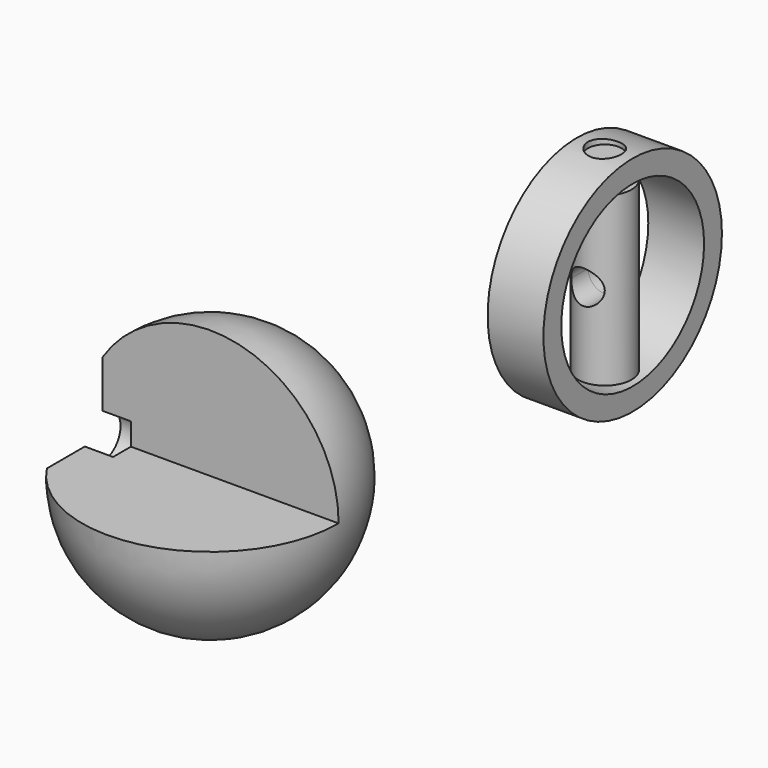
from build123d import *

# Parameters (mm, degrees)
F4_ANGLE       = 270
F5_R           = 10
F5_R_2         = 8
F6_DEPTH       = 5
F8_DEPTH       = 11
F8_DEPTH_BACK  = 25
F11_DEPTH      = 7.5
F11_DEPTH_BACK = 7.5
F12_DEPTH      = 4
F12_DEPTH_BACK = 4
F13_R          = 1.5
F14_DEPTH      = 2
F15_R          = 1.5
F16_DEPTH      = 2


# Not quite as in the source:
# - the program builds the solid bodies; features that only make, move or delete a surface that nothing else refers to are left out


with BuildPart() as f4:
    # F3 (on Front) → F4 (revolve)
    with BuildSketch(Plane.XZ):
        with BuildLine():
            Line((-7.119815331, 0), (11.5, 0))
            ThreePointArc((11.5, 0), (3.2585484641, 11.0286835981), (-9.6533672882, 6.25))
            Line((-9.6533672882, 6.25), (-9.6533672882, 2))
            Line((-9.6533672882, 2), (-7.119815331, 2))
            Line((-7.119815331, 2), (-7.119815331, 0))
        make_face()
    revolve(axis=Axis((-0.0106887892, 0, 0), (-1, 0, 0)), revolution_arc=F4_ANGLE)


with BuildPart() as f6:
    # F5 (on Right) → F6 (new body)
    with BuildSketch(Plane.YZ):
        with Locations((41.0664686725, 0)):
            Circle(F5_R)
        with Locations((41.0664686725, 0)):
            Circle(F5_R_2, mode=Mode.SUBTRACT)
    extrude(amount=F6_DEPTH)

    # F7 (on Top) → F8 (cut, two sides)
    with BuildSketch(Plane.XY) as f8_sk:
        with BuildLine():
            ThreePointArc((4, 41.0664686725), (2.5, 42.5664686725), (1, 41.0664686725))
            ThreePointArc((1, 41.0664686725), (2.5, 39.5664686725), (4, 41.0664686725))
        make_face()
    extrude(amount=-F8_DEPTH, mode=Mode.SUBTRACT)
    extrude(f8_sk.sketch, amount=F8_DEPTH_BACK, mode=Mode.SUBTRACT)


with BuildPart() as f11:
    # F7 (on Top) → F11 (new body, two sides)
    with BuildSketch(Plane.XY) as f11_sk:
        with BuildLine():
            ThreePointArc((4.9, 41.0664686725), (2.5, 43.4664686725), (0.1, 41.0664686725))
            ThreePointArc((0.1, 41.0664686725), (2.5, 38.6664686725), (4.9, 41.0664686725))
        make_face()
        with BuildLine():
            ThreePointArc((4, 41.0664686725), (2.5, 39.5664686725), (1, 41.0664686725))
            ThreePointArc((1, 41.0664686725), (2.5, 42.5664686725), (4, 41.0664686725))
        make_face(mode=Mode.SUBTRACT)
        with BuildLine():
            ThreePointArc((4, 41.0664686725), (2.5, 42.5664686725), (1, 41.0664686725))
            ThreePointArc((1, 41.0664686725), (2.5, 39.5664686725), (4, 41.0664686725))
        make_face()
    extrude(amount=F11_DEPTH)
    extrude(f11_sk.sketch, amount=-F11_DEPTH_BACK)

    # F10 (on face) → F12 (cut, two sides)
    with BuildSketch(Plane.XZ.offset(-41.0664686725)) as f12_sk:
        with BuildLine():
            ThreePointArc((1, 0), (2.5, -1.5), (4, 0))
            ThreePointArc((4, 0), (3.5606601718, 1.0606601718), (2.5, 1.5))
            Line((2.5, 1.5), (2.5, 0))
            Line((2.5, 0), (1, 0))
        make_face()
        with BuildLine():
            Line((2.5, 0), (2.5, 1.5))
            ThreePointArc((2.5, 1.5), (1.4393398282, 1.0606601718), (1, 0))
            Line((1, 0), (2.5, 0))
        make_face()
    extrude(amount=-F12_DEPTH, mode=Mode.SUBTRACT)
    extrude(f12_sk.sketch, amount=F12_DEPTH_BACK, mode=Mode.SUBTRACT)

    # F13 (on face) → F14 (join)
    with BuildSketch(Plane.XY.offset(7.5)):
        with Locations((2.5, 41.0664686725)):
            Circle(F13_R)
    extrude(amount=F14_DEPTH)

    # F15 (on face) → F16 (join)
    with BuildSketch(Plane(origin=(0, 0, -7.5), x_dir=(1, 0, 0), z_dir=(0, 0, -1))):
        with Locations((2.5, -41.0664686725)):
            Circle(F15_R)
    extrude(amount=F16_DEPTH)


solid = Compound([f4.part, f6.part, f11.part])
